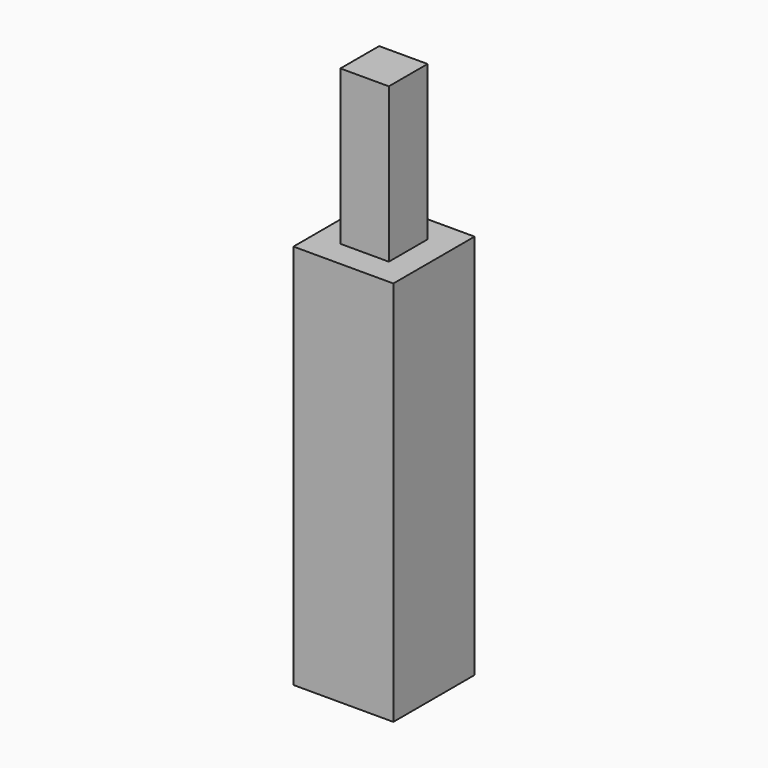
from build123d import *

# Parameters (mm, degrees)
F0_W     = 131.4967681688
F0_H     = 133.6167007685
F1_DEPTH = 508
F2_W     = 63.7412965298
F2_H     = 63.7413039804
F3_DEPTH = 203.2


# Not quite as in the source:
# - the program builds the solid bodies; features that only make, move or delete a surface that nothing else refers to are left out


with BuildPart() as f1:
    # F0 (on Top) → F1 (new body)
    with BuildSketch(Plane.XY):
        Rectangle(F0_W, F0_H)
    extrude(amount=F1_DEPTH)

    # F2 (on face) → F3 (join)
    with BuildSketch(Plane.XY.offset(508)):
        Rectangle(F2_W, F2_H)
    extrude(amount=F3_DEPTH)


solid = f1.part
